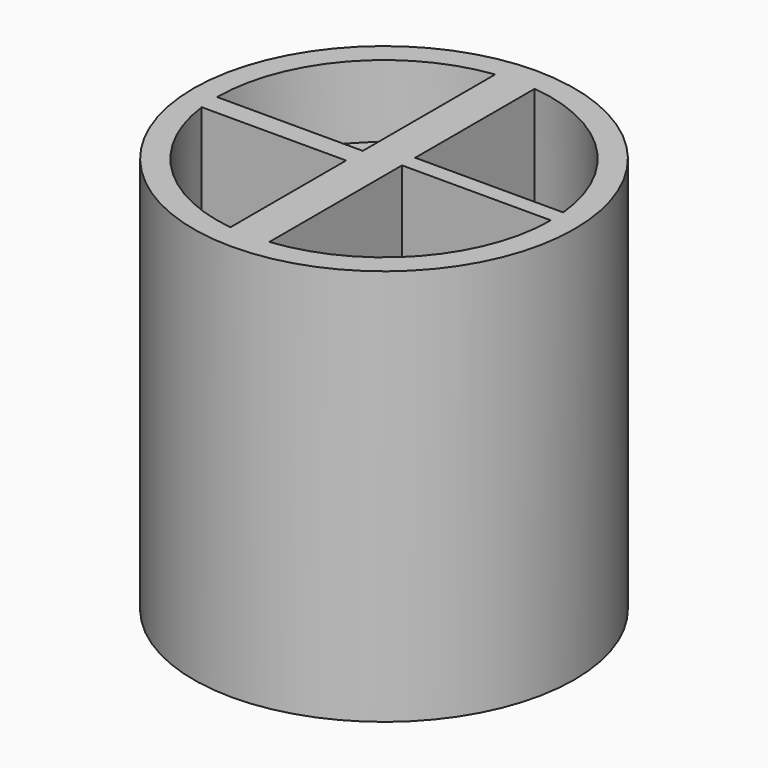
from build123d import *

# Parameters (mm, degrees)
F0_R     = 67.0773206954
F1_DEPTH = 69.85
F2_DEPTH = 6.35
F3_DEPTH = 44.45


# Not quite as in the source:
# - a feature names something its author has since deleted; it is built from what else it names


with BuildPart() as f1:
    # F0 (on Top) → F1 (new body, symmetric)
    with BuildSketch(Plane.XY):
        Circle(F0_R)
        with BuildLine():
            ThreePointArc((58.4782874441, 5.8071771637), (58.6939681668, 2.9071480599), (58.7659204727, 0))
            ThreePointArc((58.7659204727, 0), (43.7402884604, -39.2456440183), (6.3470844528, -58.4221527159))
            ThreePointArc((6.3470844528, -58.4221527159), (-0.5649559649, -58.7632047608), (-7.469161507, -58.2893217956))
            ThreePointArc((-7.469161507, -58.2893217956), (-41.5941780551, -41.5133443718), (-58.3037411026, -7.3557584547))
            ThreePointArc((-58.3037411026, -7.3557584547), (-58.6502618149, -3.6851320266), (-58.7659204727, 0))
            ThreePointArc((-58.7659204727, 0), (-44.1155616542, 38.8233258357), (-7.469161507, 58.2893217956))
            ThreePointArc((-7.469161507, 58.2893217956), (-0.5649559649, 58.7632047608), (6.3470844528, 58.4221527159))
            ThreePointArc((6.3470844528, 58.4221527159), (41.745252706, 41.3614226729), (58.4782874441, 5.8071771637))
        make_face(mode=Mode.SUBTRACT)
        with BuildLine():
            ThreePointArc((-7.469161507, -58.2893217956), (-0.5649559649, -58.7632047608), (6.3470844528, -58.4221527159))
            Line((6.3470844528, -58.4221527159), (6.3470844528, 0))
            Line((6.3470844528, 0), (6.3470844528, 5.8071771637))
            Line((6.3470844528, 5.8071771637), (6.3470844528, 58.4221527159))
            ThreePointArc((6.3470844528, 58.4221527159), (-0.5649559649, 58.7632047608), (-7.469161507, 58.2893217956))
            Line((-7.469161507, 58.2893217956), (-7.469161507, 0))
            Line((-7.469161507, 0), (-7.469161507, -7.3557584547))
            Line((-7.469161507, -7.3557584547), (-7.469161507, -58.2893217956))
        make_face()
        with BuildLine():
            Line((6.3470844528, 0), (58.7659204727, 0))
            ThreePointArc((58.7659204727, 0), (58.6939681668, 2.9071480599), (58.4782874441, 5.8071771637))
            Line((58.4782874441, 5.8071771637), (6.3470844528, 5.8071771637))
            Line((6.3470844528, 5.8071771637), (6.3470844528, 0))
        make_face()
        with BuildLine():
            ThreePointArc((-58.7659204727, 0), (-58.6502618149, -3.6851320266), (-58.3037411026, -7.3557584547))
            Line((-58.3037411026, -7.3557584547), (-7.469161507, -7.3557584547))
            Line((-7.469161507, -7.3557584547), (-7.469161507, 0))
            Line((-7.469161507, 0), (-58.7659204727, 0))
        make_face()
    extrude(amount=F1_DEPTH, both=True)

    # F0 (on Top) → F2 (join, symmetric)
    with BuildSketch(Plane.XY):
        with BuildLine():
            ThreePointArc((-58.7659204727, 0), (-58.6502618149, -3.6851320266), (-58.3037411026, -7.3557584547))
            Line((-58.3037411026, -7.3557584547), (-7.469161507, -7.3557584547))
            Line((-7.469161507, -7.3557584547), (-7.469161507, 0))
            Line((-7.469161507, 0), (-58.7659204727, 0))
        make_face()
        with BuildLine():
            Line((6.3470844528, 5.8071771637), (58.4782874441, 5.8071771637))
            ThreePointArc((58.4782874441, 5.8071771637), (41.745252706, 41.3614226729), (6.3470844528, 58.4221527159))
            Line((6.3470844528, 58.4221527159), (6.3470844528, 5.8071771637))
        make_face()
        with BuildLine():
            ThreePointArc((6.3470844528, -58.4221527159), (43.7402884604, -39.2456440183), (58.7659204727, 0))
            Line((58.7659204727, 0), (6.3470844528, 0))
            Line((6.3470844528, 0), (6.3470844528, -58.4221527159))
        make_face()
        with BuildLine():
            ThreePointArc((-58.3037411026, -7.3557584547), (-41.5941780551, -41.5133443718), (-7.469161507, -58.2893217956))
            Line((-7.469161507, -58.2893217956), (-7.469161507, -7.3557584547))
            Line((-7.469161507, -7.3557584547), (-58.3037411026, -7.3557584547))
        make_face()
    extrude(amount=F2_DEPTH, both=True)

    # F0 (on Top) → F3 (join, symmetric)
    with BuildSketch(Plane.XY):
        with BuildLine():
            Line((-7.469161507, 0), (-7.469161507, 58.2893217956))
            ThreePointArc((-7.469161507, 58.2893217956), (-44.1155616542, 38.8233258357), (-58.7659204727, 0))
            Line((-58.7659204727, 0), (-7.469161507, 0))
        make_face()
    extrude(amount=F3_DEPTH, both=True)


solid = f1.part
